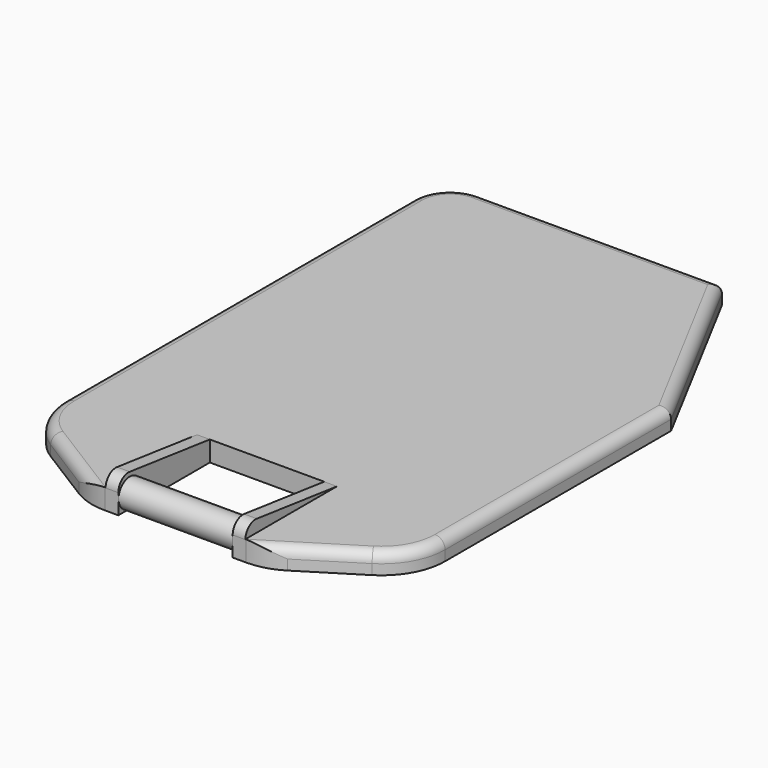
from build123d import *

# Parameters (mm, degrees)
F0_W          = 30
F0_H          = 45
F1_DEPTH      = 1.6
F2_SIZE2      = 8
F2_SIZE       = 5
F2_2_SIZE2    = 8
F2_2_SIZE     = 5
F3_R          = 3
F5_DEPTH      = 1.6
F6_W          = 11
F6_H          = 9
F7_DEPTH      = 2
F8_R          = 5
F10_DEPTH     = 1
F11_T1_DEPTH  = 6.6483183522
F13_DEPTH     = 1
F14_T1_DEPTH  = 6.6483183522
F16_T1_DEPTH  = 34.2287617925
F16_T3_DEPTH  = 24.2287617925
F16_T5_DEPTH  = 21
F16_T7_DEPTH  = 21
F16_T12_DEPTH = 8.6287617925
F16_T17_DEPTH = 8.6287617925
F16_T20_ANGLE = 57.9946167919
F16_T22_ANGLE = 90
F16_T24_ANGLE = 57.9946167919
F15_R         = 1.1066061355
F17_DEPTH     = 9


# Not quite as in the source:
# - a fillet or chamfer that OpenCascade refuses, or shapes differently, is made with other operations: its cross-section is extruded or revolved along the edge and cut away or added


with BuildPart() as f1:
    # F0 (on Top) → F1 (new body)
    with BuildSketch(Plane.XY):
        with Locations((-15, 22.5)):
            Rectangle(F0_W, F0_H)
    extrude(amount=F1_DEPTH)

    # F2
    f2_edges = [f1.edges().sort_by_distance(p)[0] for p in [
        (0, 0, 0.8),
    ]]
    f2_side = f1.faces().sort_by_distance((0, 22.5, 0.8))[0]
    chamfer(f2_edges, length=F2_SIZE, length2=F2_SIZE2, reference=f2_side)

    # F2#2
    f2_2_edges = [f1.edges().sort_by_distance(p)[0] for p in [
        (-30, 0, 0.8),
    ]]
    f2_2_side = f1.faces().sort_by_distance((-30, 22.5, 0.8))[0]
    chamfer(f2_2_edges, length=F2_2_SIZE, length2=F2_2_SIZE2, reference=f2_2_side)

    # F3
    f3_edges = [f1.edges().sort_by_distance(p)[0] for p in [
        (0, 45, 0.8),
        (-30, 45, 0.8),
    ]]
    fillet(f3_edges, radius=F3_R)

    # F4 (on face) → F5 (cut)
    with BuildSketch(Plane(origin=(0, 0, 0), x_dir=(1, 0, 0), z_dir=(0, 0, -1))):
        Polygon((0, -45), (0, -30), (-8, -45), align=None)
    extrude(amount=-F5_DEPTH, mode=Mode.SUBTRACT)

    # F6 (on face) → F7 (cut)
    with BuildSketch(Plane.XY.offset(1.6)):
        with Locations((-15, 4.5)):
            Rectangle(F6_W, F6_H)
    extrude(amount=-F7_DEPTH, mode=Mode.SUBTRACT)

    # F8
    f8_edges = [f1.edges().sort_by_distance(p)[0] for p in [
        (0, 5, 0.8),
        (-8, 0, 0.8),
        (-22, 0, 0.8),
        (-30, 5, 0.8),
    ]]
    fillet(f8_edges, radius=F8_R)

    # F9 (on face) → F10 (join)
    with BuildSketch(Plane(origin=(-9.5, 0, 0), x_dir=(0, -1, 0), z_dir=(-1, 0, 0))):
        Polygon((0, 2.7), (-9, 1.6), (-9, 0), (0, 0), align=None)
    extrude(amount=F10_DEPTH)

    # F11: fillet of radius 1 on 1 edges, made by hand

    # F11_s2 → F11_t1 (cut)
    with BuildSketch(Plane.YZ.offset(-13.3241591761)):
        with BuildLine():
            ThreePointArc((1.12131943, 2.5629498474), (0.3371725073, 2.3191084678), (0, 1.5703363296))
            Line((0, 1.5703363296), (0, 2.7))
            Line((0, 2.7), (1.12131943, 2.5629498474))
        make_face()
    extrude(amount=F11_T1_DEPTH, mode=Mode.SUBTRACT)

    # F12 (on face) → F13 (join)
    with BuildSketch(Plane.YZ.offset(-20.5)):
        Polygon((0, 2.7), (0, 0), (9, 0), (9, 1.6), align=None)
    extrude(amount=F13_DEPTH)

    # F14: fillet of radius 1 on 1 edges, made by hand

    # F14_s2 → F14_t1 (cut)
    with BuildSketch(Plane.YZ.offset(-23.3241591761)):
        with BuildLine():
            ThreePointArc((1.12131943, 2.5629498474), (0.3371725073, 2.3191084678), (0, 1.5703363296))
            Line((0, 1.5703363296), (0, 2.7))
            Line((0, 2.7), (1.12131943, 2.5629498474))
        make_face()
    extrude(amount=F14_T1_DEPTH, mode=Mode.SUBTRACT)

    # F16: fillet of radius 0.8 on 9 edges, made by hand

    # F16_s2 → F16_t1 (cut)
    with BuildSketch(Plane.XZ.offset(-42)):
        with BuildLine():
            ThreePointArc((-30, 0.8), (-29.7656854249, 1.3656854249), (-29.2, 1.6))
            Line((-29.2, 1.6), (-30, 1.6))
            Line((-30, 1.6), (-30, 0.8))
        make_face()
    extrude(amount=F16_T1_DEPTH, mode=Mode.SUBTRACT)

    # F16_s4 → F16_t3 (cut)
    with BuildSketch(Plane.XZ.offset(-32)):
        with BuildLine():
            ThreePointArc((0, 0.8), (-0.2343145751, 1.3656854249), (-0.8, 1.6))
            Line((-0.8, 1.6), (0, 1.6))
            Line((0, 1.6), (0, 0.8))
        make_face()
    extrude(amount=F16_T3_DEPTH, mode=Mode.SUBTRACT)

    # F16_s6 → F16_t5 (cut)
    with BuildSketch(Plane.YZ.offset(-27)):
        with BuildLine():
            ThreePointArc((45, 0.8), (44.7656854249, 1.3656854249), (44.2, 1.6))
            Line((44.2, 1.6), (45, 1.6))
            Line((45, 1.6), (45, 0.8))
        make_face()
    extrude(amount=F16_T5_DEPTH, mode=Mode.SUBTRACT)

    # F16_s8 → F16_t7 (cut)
    with BuildSketch(Plane(origin=(-11.5155709343, 21.5916955017, 0), x_dir=(0, 0, 1), z_dir=(-0.4705882353, 0.8823529412, 0))):
        with BuildLine():
            ThreePointArc((0.8, 14.1176470588), (1.3656854249, 13.8833324838), (1.6, 13.3176470588))
            Line((1.6, 13.3176470588), (1.6, 14.1176470588))
            Line((1.6, 14.1176470588), (0.8, 14.1176470588))
        make_face()
    extrude(amount=F16_T7_DEPTH, mode=Mode.SUBTRACT)


with BuildPart() as f16_tool10:
    # F16_s11 → F16_t12 (new body)
    with BuildSketch(Plane(origin=(-21.4702194191, 13.4188871369, 0), x_dir=(0, 0, 1), z_dir=(0.847998304, -0.52999894, 0))):
        with BuildLine():
            ThreePointArc((0.8, 11.6599766801), (1.3656854249, 11.425662105), (1.6, 10.8599766801))
            Line((1.6, 10.8599766801), (1.6, 11.6599766801))
            Line((1.6, 11.6599766801), (0.8, 11.6599766801))
        make_face()
    extrude(amount=F16_T12_DEPTH)

    split(bisect_by=Plane.YZ.offset(-20.5), keep=Keep.BOTTOM)


with BuildPart() as f1_1:
    add(f1.part)

    # F16_t9: cut F16_tool10
    add(f16_tool10.part, mode=Mode.SUBTRACT)


with BuildPart() as f16_tool15:
    # F16_s16 → F16_t17 (new body)
    with BuildSketch(Plane(origin=(-0.1028142887, -0.0642589305, 0), x_dir=(0, 0, 1), z_dir=(-0.847998304, -0.52999894, 0))):
        with BuildLine():
            ThreePointArc((0.8, 4.23999152), (1.3656854249, 4.4743060951), (1.6, 5.03999152))
            Line((1.6, 5.03999152), (1.6, 4.23999152))
            Line((1.6, 4.23999152), (0.8, 4.23999152))
        make_face()
    extrude(amount=F16_T17_DEPTH)

    split(bisect_by=Plane.YZ.offset(-9.5), keep=Keep.TOP)


with BuildPart() as f1_2:
    add(f1_1.part)

    # F16_t14: cut F16_tool15
    add(f16_tool15.part, mode=Mode.SUBTRACT)

    # F16_s19 → F16_t20 (revolve, cut)
    with BuildSketch(Plane.XZ.offset(-7.7712382075)):
        with BuildLine():
            ThreePointArc((0, 0.8), (-0.2343145751, 1.3656854249), (-0.8, 1.6))
            Line((-0.8, 1.6), (0, 1.6))
            Line((0, 1.6), (0, 0.8))
        make_face()
    revolve(axis=Axis((-5, 7.7712382075, 1.6), (0, 0, -1)), revolution_arc=F16_T20_ANGLE, mode=Mode.SUBTRACT)

    # F16_s21 → F16_t22 (revolve, cut)
    with BuildSketch(Plane.XZ.offset(-42)):
        with BuildLine():
            ThreePointArc((-30, 0.8), (-29.7656854249, 1.3656854249), (-29.2, 1.6))
            Line((-29.2, 1.6), (-30, 1.6))
            Line((-30, 1.6), (-30, 0.8))
        make_face()
    revolve(axis=Axis((-27, 42, 1.6), (0, 0, -1)), revolution_arc=F16_T22_ANGLE, mode=Mode.SUBTRACT)

    # F16_s23 → F16_t24 (revolve, cut)
    with BuildSketch(Plane(origin=(-21.4702194191, 13.4188871369, 0), x_dir=(0, 0, 1), z_dir=(0.847998304, -0.52999894, 0))):
        with BuildLine():
            ThreePointArc((0.8, 11.6599766801), (1.3656854249, 11.425662105), (1.6, 10.8599766801))
            Line((1.6, 10.8599766801), (1.6, 11.6599766801))
            Line((1.6, 11.6599766801), (0.8, 11.6599766801))
        make_face()
    revolve(axis=Axis((-25, 7.7712382075, 1.6), (0, 0, -1)), revolution_arc=F16_T24_ANGLE, mode=Mode.SUBTRACT)

    # F15 (on face) → F17 (join)
    with BuildSketch(Plane.YZ.offset(-19.5)):
        with Locations((1.125, 1.125)):
            Circle(F15_R)
    extrude(amount=F17_DEPTH)


solid = f1_2.part
